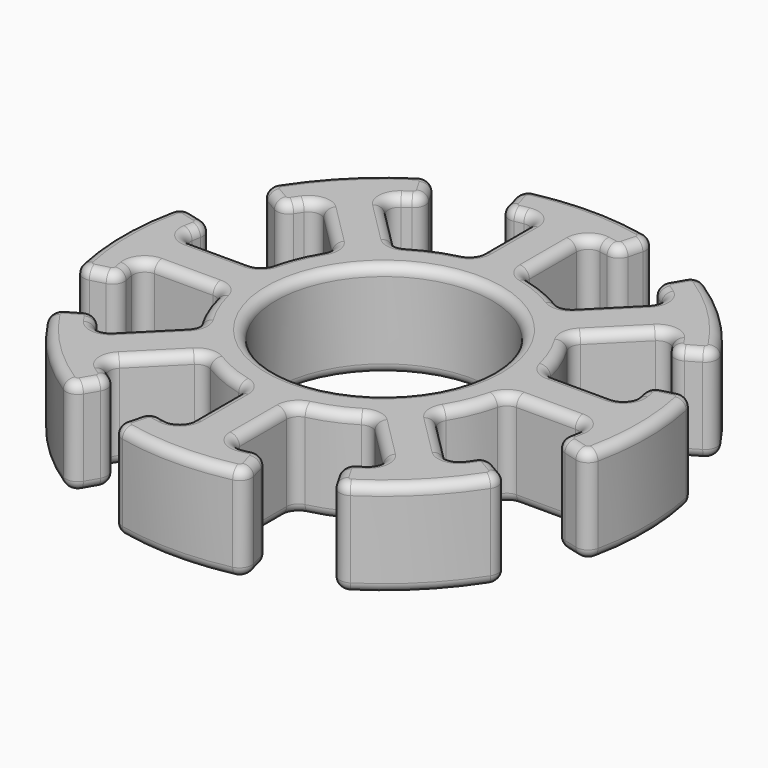
from build123d import *

# Parameters (mm, degrees)
F0_R     = 2.25
F1_DEPTH = 2
F2_R     = 0.25
F3_R     = 0.2
F4_COUNT = 8


with BuildPart() as f1:
    # F0 (on Top) → F1 (new body)
    with BuildSketch(Plane.XY):
        with BuildLine():
            Line((1.2, 4.544227), (1.404255, 5.317713))
            ThreePointArc((1.404255, 5.317713), (0, 5.5), (-1.404255, 5.317713))
            Line((-1.404255, 5.317713), (-1.2, 4.544227))
            ThreePointArc((-1.2, 4.544227), (-0.852448, 4.622049), (-0.5, 4.673329))
            Line((-0.5, 4.673329), (-0.5, 2.95804))
            ThreePointArc((-0.5, 2.95804), (0, 3), (0.5, 2.95804))
            Line((0.5, 2.95804), (0.5, 4.673329))
            ThreePointArc((0.5, 4.673329), (0.852448, 4.622049), (1.2, 4.544227))
        make_face()
        with BuildLine():
            ThreePointArc((3, 0), (2.291288, 1.936492), (0.5, 2.95804))
            ThreePointArc((0.5, 2.95804), (0, 3), (-0.5, 2.95804))
            ThreePointArc((-0.5, 2.95804), (-1.936492, -2.291288), (3, 0))
        make_face()
        Circle(F0_R, mode=Mode.SUBTRACT)
    extrude(amount=F1_DEPTH)

    # F2
    f2_edges = [f1.edges().sort_by_distance(p)[0] for p in [
        (-0.5, 4.673329, 1),
        (-1.2, 4.544227, 1),
        (-1.404255, 5.317713, 1),
        (0.5, 4.673329, 1),
        (1.2, 4.544227, 1),
        (1.404255, 5.317713, 1),
        (-0.5, 2.95804, 1),
        (0.5, 2.95804, 1),
    ]]
    fillet(f2_edges, radius=F2_R)

    # F3
    f3_edges = [f1.edges().sort_by_distance(p)[0] for p in [
        (-0.88071, 4.616747, 2),
        (-1.151703, 4.630857, 2),
        (-0.588807, 4.577436, 2),
        (-1.300561, 4.925037, 2),
        (-0.5, 3.77431, 2),
        (-1.310186, 5.264963, 2),
        (-0.553884, 3.007234, 2),
        (0, 5.5, 2),
        (0, -3, 2),
        (1.310186, 5.264963, 2),
        (0.553884, 3.007234, 2),
        (1.300561, 4.925037, 2),
        (0.5, 3.77431, 2),
        (1.151703, 4.630857, 2),
        (0.588807, 4.577436, 2),
        (0.88071, 4.616747, 2),
        (-2.25, 0, 2),
        (-0.88071, 4.616747, 0),
        (-1.151703, 4.630857, 0),
        (-0.588807, 4.577436, 0),
        (-1.300561, 4.925037, 0),
        (-0.5, 3.77431, 0),
        (-1.310186, 5.264963, 0),
        (-0.553884, 3.007234, 0),
        (0, 5.5, 0),
        (0, -3, 0),
        (1.310186, 5.264963, 0),
        (0.553884, 3.007234, 0),
        (1.300561, 4.925037, 0),
        (0.5, 3.77431, 0),
        (1.151703, 4.630857, 0),
        (0.588807, 4.577436, 0),
        (0.88071, 4.616747, 0),
        (-2.25, 0, 0),
    ]]
    fillet(f3_edges, radius=F3_R)

    # F4: F1 ×8 about axis
    f4_axis = Axis((0, 0, 2), (0, 0, 1))


with BuildPart() as f1_1:
    add(f1.part)
    for i in range(1, F4_COUNT):
        add(f1.part.rotate(f4_axis, i * 360 / F4_COUNT))


solid = f1_1.part
